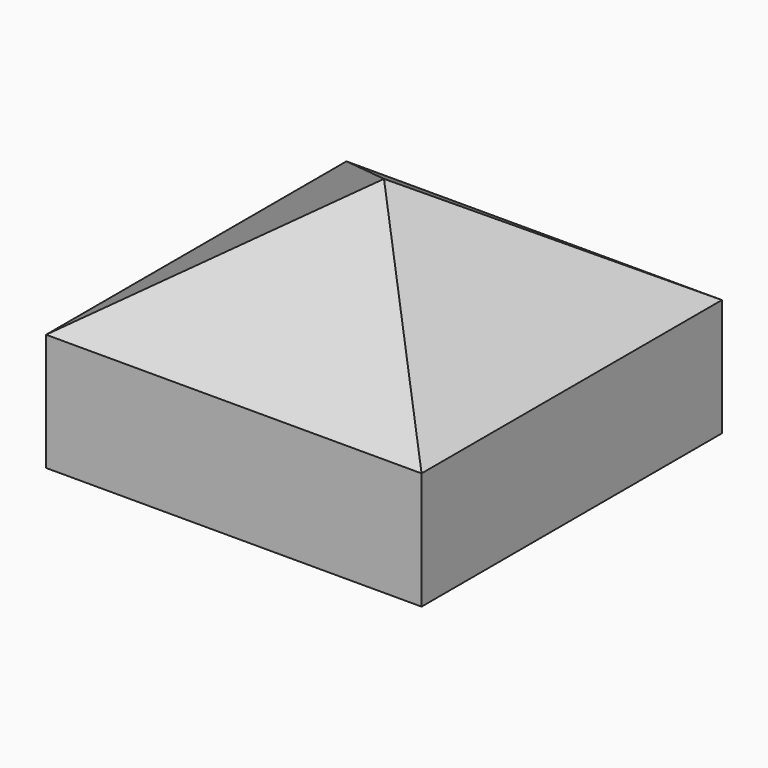
from build123d import *

# Parameters (mm, degrees)
F0_W       = 304.8
F0_H       = 304.8
F1_DEPTH   = 95.25
F1_FACE_W  = 304.8
F1_FACE_H  = 304.8
F2_DEPTH   = 101.6
F2_TAPER   = 57
F1_FACE1_W = 304.8
F1_FACE1_H = 304.8


# Not quite as in the source:
# - an extrude whose draft closes it to a point is written as a loft to that point


with BuildPart() as f1:
    # F0 (on Top) → F1 (new body)
    with BuildSketch(Plane.XY):
        with Locations((152.4, -152.4)):
            Rectangle(F0_W, F0_H)
    extrude(amount=F1_DEPTH)

    # F1_face (on face) → F2 (join)
    with BuildSketch(Plane(origin=(152.4, -152.4, 95.25), x_dir=(1, 0, 0), z_dir=(0, 0, 1))):
        Rectangle(F1_FACE_W, F1_FACE_H)
    extrude(amount=F2_DEPTH, taper=F2_TAPER)

    # F1_face1 (on face) → F3 section 0
    with BuildSketch(Plane(origin=(152.4, -152.4, 0), x_dir=(1, 0, 0), z_dir=(0, 0, -1)), mode=Mode.PRIVATE) as f3_s0:
        Rectangle(F1_FACE1_W, F1_FACE1_H)
    loft([f3_s0.sketch, Vertex(152.4, -152.4, -98.9697172033)], ruled=True)


solid = f1.part
